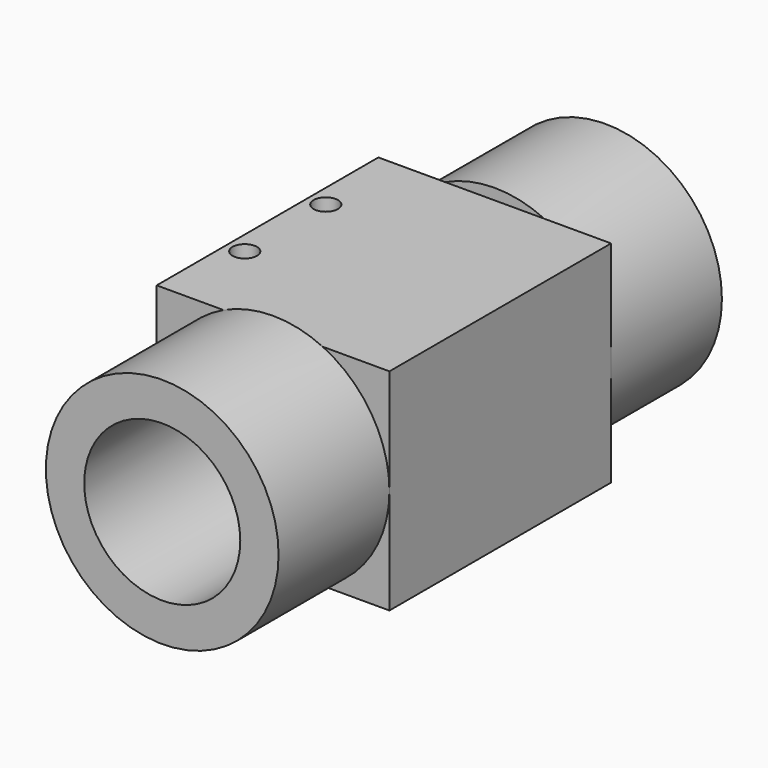
from build123d import *

# Parameters (mm, degrees)
F5_W      = 26.67
F5_H      = 26.67
F6_DEPTH  = 31.75
F7_R      = 13.335
F9_DEPTH  = 15.875
F8_R      = 13.335
F10_DEPTH = 15.875
F12_R     = 7.3025
F14_DEPTH = 63.5
F11_R     = 8.9408
F15_DEPTH = 45.72
F13_R     = 7.3025
F16_DEPTH = 63.5
F18_D     = 2.794
F19_D     = 2.794
F20_DEPTH = 1.27
F21_DEPTH = 1.27


with BuildPart() as f6:
    # F5 (on offset) → F6 (new body)
    with BuildSketch(Plane.XZ.offset(15.875)):
        Rectangle(F5_W, F5_H)
    extrude(amount=-F6_DEPTH)

    # F7 (on offset) → F9 (join)
    with BuildSketch(Plane.XZ.offset(15.875)):
        Circle(F7_R)
    extrude(amount=F9_DEPTH)

    # F8 (on offset) → F10 (join)
    with BuildSketch(Plane.XZ.offset(-15.875)):
        Circle(F8_R)
    extrude(amount=-F10_DEPTH)

    # F12 (on offset) → F14 (cut)
    with BuildSketch(Plane.XZ.offset(31.75)):
        Circle(F12_R)
    extrude(amount=-F14_DEPTH, mode=Mode.SUBTRACT)

    # F11 (on offset) → F15 (cut)
    with BuildSketch(Plane.XZ.offset(31.75)):
        Circle(F11_R)
    extrude(amount=-F15_DEPTH, mode=Mode.SUBTRACT)

    # F13 (on offset) → F16 (cut)
    with BuildSketch(Plane.XZ.offset(-31.75)):
        Circle(F13_R)
    extrude(amount=F16_DEPTH, mode=Mode.SUBTRACT)

    # F18 (through all)
    with Locations(Plane(origin=(0, 0, -13.335), x_dir=(1, 0, 0), z_dir=(0, 0, -1))):
        with Locations((-11.303, -5.8039)):
            Hole(F18_D / 2)

    # F19 (through all)
    with Locations(Plane(origin=(0, 0, -13.335), x_dir=(1, 0, 0), z_dir=(0, 0, -1))):
        with Locations((-11.303, 5.8039)):
            Hole(F19_D / 2)

    # F20 (cut): a face of the model
    f20_faces = [f6.faces().sort_by_distance(p)[0] for p in [
        (0.166086667, 0, 13.335),
    ]]
    extrude(f20_faces, amount=-F20_DEPTH, mode=Mode.SUBTRACT)

    # F21 (cut): a face of the model
    f21_faces = [f6.faces().sort_by_distance(p)[0] for p in [
        (0.166086667, 0, -13.335),
    ]]
    extrude(f21_faces, amount=-F21_DEPTH, mode=Mode.SUBTRACT)


solid = f6.part
